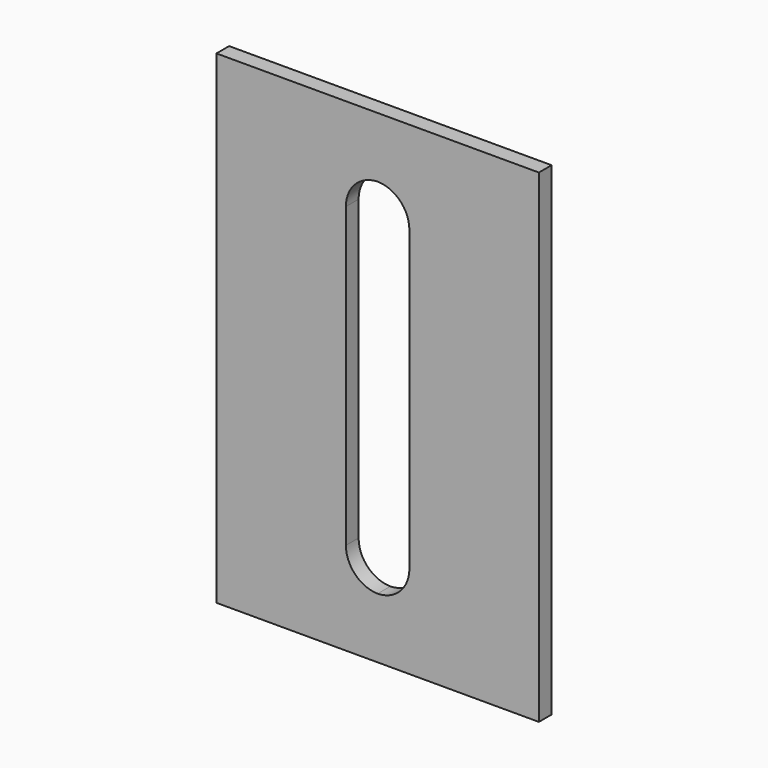
from build123d import *

# Parameters (mm, degrees)
F0_W        = 101.6
F0_H        = 152.4
F0_W_2      = 20
F0_H_2      = 114.3
F1_DEPTH    = 5
F2_T1_DEPTH = 5


# Not quite as in the source:
# - a fillet or chamfer that OpenCascade refuses, or shapes differently, is made with other operations: its cross-section is extruded or revolved along the edge and cut away or added


with BuildPart() as f1:
    # F0 (on Front) → F1 (new body)
    with BuildSketch(Plane.XZ):
        Rectangle(F0_W, F0_H)
        Rectangle(F0_W_2, F0_H_2, mode=Mode.SUBTRACT)
    extrude(amount=F1_DEPTH)

    # F2: fillet of radius 10.16 on 4 edges, made by hand

    # F2_s2 → F2_t1 (join)
    with BuildSketch(Plane.XZ):
        with BuildLine():
            ThreePointArc((-10, 46.99), (-7.0242048969, 54.1742048969), (0.16, 57.15))
            Line((0.16, 57.15), (-10, 57.15))
            Line((-10, 57.15), (-10, 46.99))
        make_face()
        with BuildLine():
            ThreePointArc((10, 46.99), (7.0242048969, 54.1742048969), (-0.16, 57.15))
            Line((-0.16, 57.15), (10, 57.15))
            Line((10, 57.15), (10, 46.99))
        make_face()
        with BuildLine():
            ThreePointArc((10, -46.99), (7.0242048969, -54.1742048969), (-0.16, -57.15))
            Line((-0.16, -57.15), (10, -57.15))
            Line((10, -57.15), (10, -46.99))
        make_face()
        with BuildLine():
            ThreePointArc((0.16, -57.15), (-7.0242048969, -54.1742048969), (-10, -46.99))
            Line((-10, -46.99), (-10, -57.15))
            Line((-10, -57.15), (0.16, -57.15))
        make_face()
    extrude(amount=F2_T1_DEPTH)


solid = f1.part
